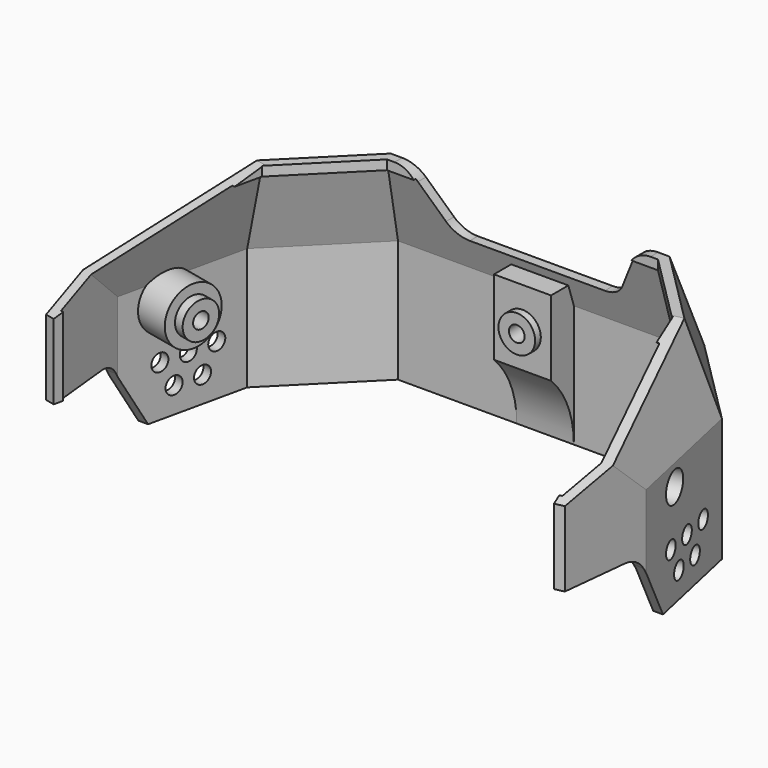
from build123d import *

# Parameters (mm, degrees)
F1_DEPTH  = 44
F2_SIZE2  = 6
F2_SIZE   = 18
F3_SIZE2  = 18
F3_SIZE   = 6
F4_SIZE2  = 6
F4_SIZE   = 18
F5_T      = -2
F7_DEPTH  = 6
F8_DEPTH  = 6
F9_R      = 3.85
F10_DEPTH = 1.5
F11_R     = 1.65
F12_DEPTH = 9.5
F14_DEPTH = 8
F16_DEPTH = 8
F18_DEPTH = 58.1260003197
F19_DEPTH = 58.1260003197
F21_DEPTH = 8
F22_R     = 5
F23_R     = 4
F24_DEPTH = 1
F25_SIZE  = 0.99999
F27_DEPTH = 1
F28_SIZE  = 0.99999
F30_DEPTH = 1
F31_SIZE  = 0.99999
F32_R     = 6
F33_DEPTH = 7
F34_R     = 6
F35_DEPTH = 7
F36_R     = 3.85
F37_DEPTH = 2
F38_R     = 3.85
F39_DEPTH = 2
F40_R     = 1.65
F41_DEPTH = 11
F42_R     = 1.65
F43_DEPTH = 11
F44_R     = 3.2
F45_DEPTH = 4
F46_R     = 3.2
F47_DEPTH = 4
F48_R     = 1.8
F49_DEPTH = 2
F50_R     = 1.8
F51_DEPTH = 2
F52_R     = 5


# Not quite as in the source:
# - a fillet or chamfer is up to 0.001 mm smaller than in the source, because OpenCascade refuses the exact size


with BuildPart() as f1:
    # F0 (on Top) → F1 (new body)
    with BuildSketch(Plane.XY):
        Polygon((-43.0871382073, 49.3898122897), (-28.476950497, 64), (28.476950497, 64), (43.0871382073, 49.3898122897), (52.5625825511, 6.5608048757), (60.3737020635, 8.2889287028), (50.394148284, 53.3965107119), (31.7906589959, 72), (-31.7906589959, 72), (-50.394148284, 53.3965107119), (-60.3737020635, 8.2889287028), (-52.5625825511, 6.5608048757), align=None)
    extrude(amount=F1_DEPTH)

    # F2
    f2_edges = [f1.edges().sort_by_distance(p)[0] for p in [
        (-55.383925, 30.84272, 44),
        (-41.092404, 62.698255, 44),
        (0, 72, 44),
        (41.092404, 62.698255, 44),
        (55.383925, 30.84272, 44),
    ]]
    chamfer(f2_edges, length=F2_SIZE, length2=F2_SIZE2)

    # F3
    f3_edges = [f1.edges().sort_by_distance(p)[0] for p in [
        (-60.373702, 8.288929, 13),
    ]]
    f3_side = f1.faces().sort_by_distance((-56.114283, 7.346579, 19.100671))[0]
    chamfer(f3_edges, length=F3_SIZE, length2=F3_SIZE2, reference=f3_side)

    # F4
    f4_edges = [f1.edges().sort_by_distance(p)[0] for p in [
        (60.373702, 8.288929, 13),
    ]]
    f4_side = f1.faces().sort_by_distance((55.383925, 30.84272, 13))[0]
    chamfer(f4_edges, length=F4_SIZE, length2=F4_SIZE2, reference=f4_side)

    # F5
    f5_openings = [f1.faces().sort_by_distance(p)[0] for p in [
        (0, 64, 22),
        (-35.782044, 56.694906, 22),
        (-47.82486, 27.975309, 22),
        (35.782044, 56.694906, 22),
        (47.82486, 27.975309, 22),
        (52.165057, 39.348209, 0),
    ]]
    offset(amount=F5_T, openings=f5_openings)

    # F6 (on Right) → F7 (join)
    with BuildSketch(Plane.YZ):
        with BuildLine():
            Line((70, 0), (70, 25.6754446797))
            Line((70, 25.6754446797), (68.5443115599, 30.04251))
            Line((68.5443115599, 30.04251), (64, 30.04251))
            Line((64, 30.04251), (64, 14.24251))
            ThreePointArc((64, 14.24251), (68.4387704324, 7.7273716602), (70, 0))
        make_face()
    extrude(amount=F7_DEPTH)

    # F6 (on Right) → F8 (join)
    with BuildSketch(Plane.YZ):
        with BuildLine():
            Line((70, 0), (70, 25.6754446797))
            Line((70, 25.6754446797), (68.5443115599, 30.04251))
            Line((68.5443115599, 30.04251), (64, 30.04251))
            Line((64, 30.04251), (64, 14.24251))
            ThreePointArc((64, 14.24251), (68.4387704324, 7.7273716602), (70, 0))
        make_face()
    extrude(amount=-F8_DEPTH)

    # F9 (on face) → F10 (join)
    with BuildSketch(Plane.XZ.offset(-64)):
        with Locations((0, 21.6)):
            Circle(F9_R)
    extrude(amount=F10_DEPTH)

    # F11 (on face) → F12 (cut, through all)
    with BuildSketch(Plane.XZ.offset(-62.5)):
        with Locations((0, 21.6)):
            Circle(F11_R)
    extrude(amount=-F12_DEPTH, mode=Mode.SUBTRACT)

    # F13 (on face) → F14 (cut, through all)
    with BuildSketch(Plane(origin=(59.3047651207, 13.1205235693, 0), x_dir=(-0.2160154784, 0.9763899391, 0), z_dir=(0.9763899391, 0.2160154784, 0))):
        Polygon((-4.9484275423, 44), (-4.9484275423, 30), (39.4996452273, 44), align=None)
    extrude(amount=-F14_DEPTH, mode=Mode.SUBTRACT)

    # F15 (on face) → F16 (cut, through all)
    with BuildSketch(Plane(origin=(-59.3047651207, 13.1205235693, 0), x_dir=(-0.2160154784, -0.9763899391, 0), z_dir=(-0.9763899391, 0.2160154784, 0))):
        Polygon((4.9484275423, 44), (-39.4996452273, 44), (4.9484275423, 30), align=None)
    extrude(amount=-F16_DEPTH, mode=Mode.SUBTRACT)

    # F17 (on Right) → F18 (cut, up to face)
    with BuildSketch(Plane.YZ):
        Polygon((6.5608048757, 0), (32, 0), (23.8016261775, 14.2), (6.5608048757, 14.2), align=None)
    extrude(amount=-F18_DEPTH, mode=Mode.SUBTRACT)

    # F17 (on Right) → F19 (cut, up to face)
    with BuildSketch(Plane.YZ):
        Polygon((6.5608048757, 0), (32, 0), (23.8016261775, 14.2), (6.5608048757, 14.2), align=None)
    extrude(amount=F19_DEPTH, mode=Mode.SUBTRACT)

    # F20 (on face) → F21 (cut, through all)
    with BuildSketch(Plane(origin=(0, 72, 0), x_dir=(-1, 0, 0), z_dir=(0, 1, 0))):
        Polygon((24, 44), (-24, 44), (-17.0717967697, 32), (17.0717967697, 32), align=None)
    extrude(amount=-F21_DEPTH, mode=Mode.SUBTRACT)

    # F22
    f22_edges = [f1.edges().sort_by_distance(p)[0] for p in [
        (17.071797, 68.945907, 32),
        (-17.071797, 68.945907, 32),
        (24, 65, 44),
        (-24, 65, 44),
    ]]
    fillet(f22_edges, radius=F22_R)

    # F23 (on face) → F24 (cut)
    with BuildSketch(Plane(origin=(0, 72, 0), x_dir=(-1, 0, 0), z_dir=(0, 1, 0))):
        with BuildLine():
            ThreePointArc((-21.7906589959, 21), (-25.3261929019, 19.5355339059), (-26.7906589959, 16))
            Line((-26.7906589959, 16), (-26.7906589959, 10))
            ThreePointArc((-26.7906589959, 10), (-25.3261929019, 6.4644660941), (-21.7906589959, 5))
            Line((-21.7906589959, 5), (21.7906589959, 5))
            ThreePointArc((21.7906589959, 5), (25.3261929019, 6.4644660941), (26.7906589959, 10))
            Line((26.7906589959, 10), (26.7906589959, 16))
            ThreePointArc((26.7906589959, 16), (25.3261929019, 19.5355339059), (21.7906589959, 21))
            Line((21.7906589959, 21), (12.8312119459, 21))
            ThreePointArc((12.8312119459, 21), (10.0925991584, 20.1833001327), (8.2486362509, 18))
            ThreePointArc((8.2486362509, 18), (0, 12.6), (-8.2486362509, 18))
            ThreePointArc((-8.2486362509, 18), (-10.0925991584, 20.1833001327), (-12.8312119459, 21))
            Line((-12.8312119459, 21), (-21.7906589959, 21))
        make_face()
        with BuildLine():
            ThreePointArc((-22.3832435079, 14.6220146604), (-23.1686443356, 16.5925845119), (-21.198074484, 17.3779853396))
            Line((-21.198074484, 17.3779853396), (-7.245782665, 11.3779853396))
            ThreePointArc((-7.245782665, 11.3779853396), (-6.4603818373, 9.4074154881), (-8.4309516888, 8.6220146604))
            Line((-8.4309516888, 8.6220146604), (-22.3832435079, 14.6220146604))
        make_face(mode=Mode.SUBTRACT)
        with BuildLine():
            Line((7.245782665, 11.3779853396), (21.198074484, 17.3779853396))
            ThreePointArc((21.198074484, 17.3779853396), (23.1686443356, 16.5925845119), (22.3832435079, 14.6220146604))
            Line((22.3832435079, 14.6220146604), (8.4309516888, 8.6220146604))
            ThreePointArc((8.4309516888, 8.6220146604), (6.4603818373, 9.4074154881), (7.245782665, 11.3779853396))
        make_face(mode=Mode.SUBTRACT)
        with Locations((0, 21.6)):
            Circle(F23_R)
    extrude(amount=-F24_DEPTH, mode=Mode.SUBTRACT)

    # F25 (size 1 in the source; OpenCascade refuses exactly that, so slightly less here)
    f25_edges = [f1.edges().sort_by_distance(p)[0] for p in [
        (0, 71, 12.6),
        (15.407098, 71, 11.622015),
        (-15.407098, 71, 11.622015),
        (4, 71, 21.6),
    ]]
    chamfer(f25_edges, length=F25_SIZE)

    # F26 (on face) → F27 (cut)
    with BuildSketch(Plane(origin=(51.895329498, 51.895329498, 0), x_dir=(-0.7071067812, 0.7071067812, 0), z_dir=(0.7071067812, 0.7071067812, 0))):
        with BuildLine():
            Line((18.432297691, 21), (12.1229908323, 21))
            ThreePointArc((12.1229908323, 21), (8.5874569264, 19.5355339059), (7.1229908323, 16))
            Line((7.1229908323, 16), (7.1229908323, 10))
            ThreePointArc((7.1229908323, 10), (8.5874569264, 6.4644660941), (12.1229908323, 5))
            Line((12.1229908323, 5), (18.432297691, 5))
            ThreePointArc((18.432297691, 5), (21.9678315969, 6.4644660941), (23.432297691, 10))
            Line((23.432297691, 10), (23.432297691, 16))
            ThreePointArc((23.432297691, 16), (21.9678315969, 19.5355339059), (18.432297691, 21))
        make_face()
    extrude(amount=-F27_DEPTH, mode=Mode.SUBTRACT)

    # F28 (size 1 in the source; OpenCascade refuses exactly that, so slightly less here)
    f28_edges = [f1.edges().sort_by_distance(p)[0] for p in [
        (45.115974, 57.260472, 19.535534),
    ]]
    chamfer(f28_edges, length=F28_SIZE)

    # F29 (on face) → F30 (cut)
    with BuildSketch(Plane(origin=(-51.895329498, 51.895329498, 0), x_dir=(-0.7071067812, -0.7071067812, 0), z_dir=(-0.7071067812, 0.7071067812, 0))):
        with BuildLine():
            Line((-12.1229908323, 21), (-18.432297691, 21))
            ThreePointArc((-18.432297691, 21), (-21.9678315969, 19.5355339059), (-23.432297691, 16))
            Line((-23.432297691, 16), (-23.432297691, 10))
            ThreePointArc((-23.432297691, 10), (-21.9678315969, 6.4644660941), (-18.432297691, 5))
            Line((-18.432297691, 5), (-12.1229908323, 5))
            ThreePointArc((-12.1229908323, 5), (-8.5874569264, 6.4644660941), (-7.1229908323, 10))
            Line((-7.1229908323, 10), (-7.1229908323, 16))
            ThreePointArc((-7.1229908323, 16), (-8.5874569264, 19.5355339059), (-12.1229908323, 21))
        make_face()
    extrude(amount=-F30_DEPTH, mode=Mode.SUBTRACT)

    # F31 (size 1 in the source; OpenCascade refuses exactly that, so slightly less here)
    f31_edges = [f1.edges().sort_by_distance(p)[0] for p in [
        (-35.65462, 66.721825, 19.535534),
    ]]
    chamfer(f31_edges, length=F31_SIZE)

    # F32 (on face) → F33 (join)
    with BuildSketch(Plane(origin=(-57.3519852426, 12.6884926125, 0), x_dir=(0.2160154784, 0.9763899391, 0), z_dir=(0.9763899391, -0.2160154784, 0))):
        with Locations((23.6515697905, 21.6)):
            Circle(F32_R)
    extrude(amount=F33_DEPTH)

    # F34 (on face) → F35 (join)
    with BuildSketch(Plane(origin=(57.3519852426, 12.6884926125, 0), x_dir=(0.2160154784, -0.9763899391, 0), z_dir=(-0.9763899391, -0.2160154784, 0))):
        with Locations((-23.6515697905, 21.6)):
            Circle(F34_R)
    extrude(amount=F35_DEPTH)

    # F36 (on face) → F37 (join)
    with BuildSketch(Plane(origin=(50.5172556692, 11.1763842638, 0), x_dir=(0.2160154784, -0.9763899391, 0), z_dir=(-0.9763899391, -0.2160154784, 0))):
        with Locations((-23.6515697905, 21.6)):
            Circle(F36_R)
    extrude(amount=F37_DEPTH)

    # F38 (on face) → F39 (join)
    with BuildSketch(Plane(origin=(-50.5172556692, 11.1763842638, 0), x_dir=(0.2160154784, 0.9763899391, 0), z_dir=(0.9763899391, -0.2160154784, 0))):
        with Locations((23.6515697905, 21.6)):
            Circle(F38_R)
    extrude(amount=F39_DEPTH)

    # F40 (on face) → F41 (cut, through all)
    with BuildSketch(Plane(origin=(48.5644757911, 10.744353307, 0), x_dir=(0.2160154784, -0.9763899391, 0), z_dir=(-0.9763899391, -0.2160154784, 0))):
        with Locations((-23.6515697905, 21.6)):
            Circle(F40_R)
    extrude(amount=-F41_DEPTH, mode=Mode.SUBTRACT)

    # F42 (on face) → F43 (cut, through all)
    with BuildSketch(Plane(origin=(-48.5644757911, 10.744353307, 0), x_dir=(0.2160154784, 0.9763899391, 0), z_dir=(0.9763899391, -0.2160154784, 0))):
        with Locations((23.6515697905, 21.6)):
            Circle(F42_R)
    extrude(amount=-F43_DEPTH, mode=Mode.SUBTRACT)

    # F44 (on face) → F45 (cut)
    with BuildSketch(Plane(origin=(-59.3047651207, 13.1205235693, 0), x_dir=(-0.2160154784, -0.9763899391, 0), z_dir=(-0.9763899391, 0.2160154784, 0))):
        with Locations((-23.6515697905, 21.6)):
            Circle(F44_R)
    extrude(amount=-F45_DEPTH, mode=Mode.SUBTRACT)

    # F46 (on face) → F47 (cut)
    with BuildSketch(Plane(origin=(59.3047651207, 13.1205235693, 0), x_dir=(-0.2160154784, 0.9763899391, 0), z_dir=(0.9763899391, 0.2160154784, 0))):
        with Locations((23.6515697905, 21.6)):
            Circle(F46_R)
    extrude(amount=-F47_DEPTH, mode=Mode.SUBTRACT)

    # F48 (on face) → F49 (cut, through all)
    with BuildSketch(Plane(origin=(59.3047651207, 13.1205235693, 0), x_dir=(-0.2160154784, 0.9763899391, 0), z_dir=(0.9763899391, 0.2160154784, 0))):
        with Locations((22.2498997905, 10.6279545047)):
            Circle(F48_R)
        with Locations((28.2498997905, 10.6279545047)):
            Circle(F48_R)
        with Locations((34.2498997905, 10.6279545047)):
            Circle(F48_R)
        with Locations((25.2498997905, 5.431802082)):
            Circle(F48_R)
        with Locations((31.2498997905, 5.431802082)):
            Circle(F48_R)
    extrude(amount=-F49_DEPTH, mode=Mode.SUBTRACT)

    # F50 (on face) → F51 (cut, through all)
    with BuildSketch(Plane(origin=(-59.3047651207, 13.1205235693, 0), x_dir=(-0.2160154784, -0.9763899391, 0), z_dir=(-0.9763899391, 0.2160154784, 0))):
        with Locations((-34.2498997905, 10.6279545043)):
            Circle(F50_R)
        with Locations((-31.2498997905, 5.4318020816)):
            Circle(F50_R)
        with Locations((-28.2498997905, 10.6279545043)):
            Circle(F50_R)
        with Locations((-25.2498997905, 5.4318020816)):
            Circle(F50_R)
        with Locations((-22.2498997905, 10.6279545043)):
            Circle(F50_R)
    extrude(amount=-F51_DEPTH, mode=Mode.SUBTRACT)

    # F52
    f52_edges = [f1.edges().sort_by_distance(p)[0] for p in [
        (55.264692, 23.801626, 14.2),
        (-55.264692, 23.801626, 14.2),
    ]]
    fillet(f52_edges, radius=F52_R)


solid = f1.part
